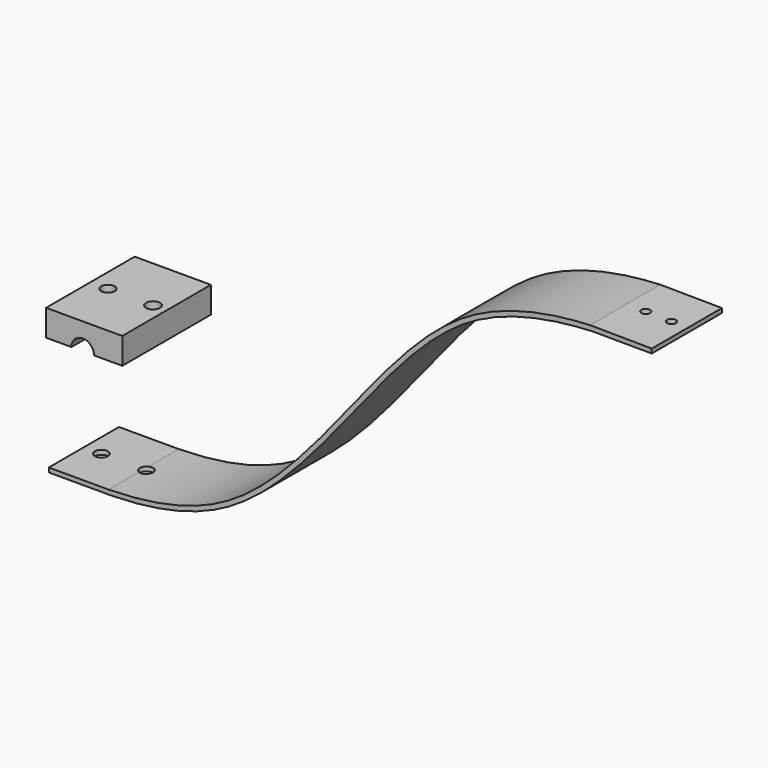
from build123d import *

# Parameters (mm, degrees)
F2_DEPTH  = 31.75
F3_R      = 1.5875
F4_DEPTH  = 2.54
F5_R      = 2.38125
F6_DEPTH  = 2.54
F7_W      = 27.578599751
F7_H      = 40.0851694867
F8_DEPTH  = 9.525
F9_R      = 2.4220384901
F9_R_2    = 2.5148035407
F10_DEPTH = 25.4
F12_DEPTH = 50.8


# Not quite as in the source:
# - the program builds the solid bodies; features that only make, move or delete a surface that nothing else refers to are left out


with BuildPart() as f2:
    # F0 (on Front) → F2 (new body)
    with BuildSketch(Plane.XZ):
        with BuildLine():
            Line((-109.7734197974, -54.4999252498), (-87.1213535286, -54.4999252498))
            add(Edge.make_bspline(
                [(-87.1213535286, -54.4999252498), (-72.0730019908, -54.2105347145), (-39.612358699, -48.6311111585), (0.2764524513, -0.055323172), (38.5858327695, 48.8342903772), (73.8190934908, 53.859632643), (87.1213535286, 54.4508459553)],
                knots=[0, 0, 0, 0, 0.230298298, 0.5000152925, 0.7697322871, 1, 1, 1, 1], degree=3))
            Line((87.1213535286, 54.4508459553), (108.4502488375, 54.3554909527))
            Line((108.4502488375, 54.3554909527), (108.4502488375, 55.9429909527))
            Line((108.4502488375, 55.9429909527), (86.1265237905, 56.1496154059))
            add(Edge.make_bspline(
                [(-88.1161832666, -52.9124252498), (-73.0779283777, -52.6232288803), (-40.5831653258, -47.3903123555), (-0.7292490562, 1.3961196705), (37.624911948, 50.0240186994), (72.8130684815, 55.5579045244), (86.1265237905, 56.1496154059)],
                knots=[0, 0, 0, 0, 0.23014378, 0.4998411361, 0.7695384922, 1, 1, 1, 1], degree=3))
            Line((-88.1161832666, -52.9124252498), (-109.7734197974, -52.9124252498))
            Line((-109.7734197974, -52.9124252498), (-109.7734197974, -54.4999252498))
        make_face()
    extrude(amount=F2_DEPTH)

    # F3 (on face) → F4 (cut)
    with BuildSketch(Plane(origin=(0.5270442453, 0, 56.9419090581), x_dir=(0.9999571676, 0, -0.0092554268), z_dir=(0.0092554268, 0, 0.9999571676))):
        with Locations((92.5925821066, -15.2800846845)):
            Circle(F3_R)
        with Locations((101.9724830985, -15.4172424227)):
            Circle(F3_R)
    extrude(amount=-F4_DEPTH, mode=Mode.SUBTRACT)

    # F5 (on face) → F6 (cut)
    with BuildSketch(Plane(origin=(0, 0, -54.4999252498), x_dir=(1, 0, 0), z_dir=(0, 0, -1))):
        with Locations((-103.4234197974, 15.875)):
            Circle(F5_R)
        with Locations((-87.1213535286, 15.875)):
            Circle(F5_R)
    extrude(amount=-F6_DEPTH, mode=Mode.SUBTRACT)


with BuildPart() as f8:
    # F7 (on Top) → F8 (new body)
    with BuildSketch(Plane.XY):
        with Locations((-94.1408313811, -15.2323641814)):
            Rectangle(F7_W, F7_H)
    extrude(amount=-F8_DEPTH)

    # F9 (on face) → F10 (cut)
    with BuildSketch(Plane(origin=(0, 0, -9.525), x_dir=(1, 0, 0), z_dir=(0, 0, -1))):
        with Locations((-101.5801312566, 15.2303794381)):
            Circle(F9_R)
        with Locations((-85.2733312566, 15.2303794381)):
            Circle(F9_R_2)
    extrude(amount=-F10_DEPTH, mode=Mode.SUBTRACT)

    # F11 (on face) → F12 (cut)
    with BuildSketch(Plane.XZ.offset(35.2749489248)):
        with BuildLine():
            Line((-98.7523206457, -9.525), (-90.5765137688, -9.525))
            ThreePointArc((-90.5765137688, -9.525), (-94.6644172072, -5.4370965615), (-98.7523206457, -9.525))
        make_face()
        with BuildLine():
            ThreePointArc((-98.7523206457, -9.525), (-94.6644172072, -13.6129034385), (-90.5765137688, -9.525))
            Line((-90.5765137688, -9.525), (-98.7523206457, -9.525))
        make_face()
    extrude(amount=-F12_DEPTH, mode=Mode.SUBTRACT)


solid = Compound([f2.part, f8.part])
